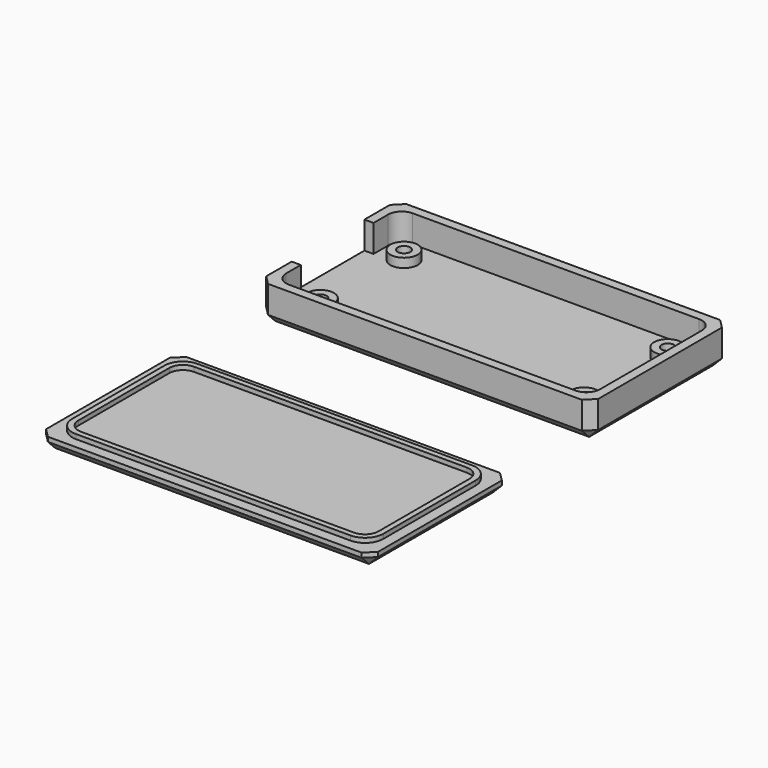
from build123d import *

# Parameters (mm, degrees)
F0_W     = 65
F0_H     = 30
F0_R     = 3
F0_R_2   = 1.375
F0_W_2   = 2
F0_H_2   = 20
F1_DEPTH = 2
F2_DEPTH = 4
F3_DEPTH = 8
F4_R     = 3
F5_SIZE  = 1.99999
F6_SIZE  = 1.7
F7_W     = 73
F7_H     = 38
F7_W_2   = 68.4
F7_H_2   = 33.4
F7_W_3   = 66
F7_H_3   = 31
F7_W_4   = 65
F7_H_4   = 30
F8_DEPTH = 3
F9_DEPTH = 4
F10_R    = 3
F11_R    = 4
F12_SIZE = 2


# Not quite as in the source:
# - a fillet or chamfer is up to 0.001 mm smaller than in the source, because OpenCascade refuses the exact size


with BuildPart() as f1:
    # F0 (on Top) → F1 (new body)
    with BuildSketch(Plane.XY):
        Polygon((-34.5, 10), (-34.5, 17), (34.5, 17), (34.5, -17), (-34.5, -17), (-34.5, -10), (-36.5, -10), (-36.5, -19), (36.5, -19), (36.5, 19), (-36.5, 19), (-36.5, 10), align=None)
        Polygon((34.5, 17), (-34.5, 17), (-34.5, 10), (-34.5, -10), (-34.5, -17), (34.5, -17), align=None)
        Rectangle(F0_W, F0_H, mode=Mode.SUBTRACT)
        Rectangle(F0_W, F0_H)
        with Locations((-29, -11.5)):
            Circle(F0_R, mode=Mode.SUBTRACT)
        with Locations((29, -11.5)):
            Circle(F0_R, mode=Mode.SUBTRACT)
        with Locations((-29, 11.5)):
            Circle(F0_R, mode=Mode.SUBTRACT)
        with Locations((29, 11.5)):
            Circle(F0_R, mode=Mode.SUBTRACT)
        with Locations((-29, 11.5)):
            Circle(F0_R)
        with Locations((-29, 11.5)):
            Circle(F0_R_2, mode=Mode.SUBTRACT)
        with Locations((29, 11.5)):
            Circle(F0_R)
        with Locations((29, 11.5)):
            Circle(F0_R_2, mode=Mode.SUBTRACT)
        with Locations((29, -11.5)):
            Circle(F0_R)
        with Locations((29, -11.5)):
            Circle(F0_R_2, mode=Mode.SUBTRACT)
        with Locations((-29, -11.5)):
            Circle(F0_R)
        with Locations((-29, -11.5)):
            Circle(F0_R_2, mode=Mode.SUBTRACT)
        with Locations((-35.5, 0)):
            Rectangle(F0_W_2, F0_H_2)
    extrude(amount=F1_DEPTH)

    # F0 (on Top) → F2 (join)
    with BuildSketch(Plane.XY):
        with Locations((-29, -11.5)):
            Circle(F0_R)
        with Locations((-29, -11.5)):
            Circle(F0_R_2, mode=Mode.SUBTRACT)
        with Locations((-29, 11.5)):
            Circle(F0_R)
        with Locations((-29, 11.5)):
            Circle(F0_R_2, mode=Mode.SUBTRACT)
        with Locations((29, -11.5)):
            Circle(F0_R)
        with Locations((29, -11.5)):
            Circle(F0_R_2, mode=Mode.SUBTRACT)
        with Locations((29, 11.5)):
            Circle(F0_R)
        with Locations((29, 11.5)):
            Circle(F0_R_2, mode=Mode.SUBTRACT)
    extrude(amount=F2_DEPTH)

    # F0 (on Top) → F3 (join)
    with BuildSketch(Plane.XY):
        Polygon((-34.5, 10), (-34.5, 17), (34.5, 17), (34.5, -17), (-34.5, -17), (-34.5, -10), (-36.5, -10), (-36.5, -19), (36.5, -19), (36.5, 19), (-36.5, 19), (-36.5, 10), align=None)
    extrude(amount=F3_DEPTH)

    # F4
    f4_edges = [f1.edges().sort_by_distance(p)[0] for p in [
        (-34.5, 17, 5),
        (-34.5, -17, 5),
        (34.5, -17, 5),
        (34.5, 17, 5),
    ]]
    fillet(f4_edges, radius=F4_R)

    # F5 (size 2 in the source; OpenCascade refuses exactly that, so slightly less here)
    f5_edges = [f1.edges().sort_by_distance(p)[0] for p in [
        (36.5, -19, 4),
        (36.5, 19, 4),
        (-36.5, 19, 4),
        (-36.5, -19, 4),
        (0, -19, 0),
        (-36.5, 0, 0),
        (0, 19, 0),
        (36.5, 0, 0),
    ]]
    chamfer(f5_edges, length=F5_SIZE)

    # F6
    f6_edges = [f1.edges().sort_by_distance(p)[0] for p in [
        (27.625, 11.5, 0),
        (27.625, -11.5, 0),
        (-30.375, -11.5, 0),
        (-30.375, 11.5, 0),
    ]]
    chamfer(f6_edges, length=F6_SIZE)


with BuildPart() as f8:
    # F7 (on Top) → F8 (new body)
    with BuildSketch(Plane.XY):
        with Locations((0, -60.494761914)):
            Rectangle(F7_W, F7_H)
        with Locations((0, -60.494761914)):
            Rectangle(F7_W_2, F7_H_2, mode=Mode.SUBTRACT)
        with Locations((0, -60.494761914)):
            Rectangle(F7_W_2, F7_H_2)
        with Locations((0, -60.494761914)):
            Rectangle(F7_W_3, F7_H_3, mode=Mode.SUBTRACT)
        with Locations((0, -60.494761914)):
            Rectangle(F7_W_3, F7_H_3)
        with Locations((0, -60.494761914)):
            Rectangle(F7_W_4, F7_H_4, mode=Mode.SUBTRACT)
        with Locations((0, -60.494761914)):
            Rectangle(F7_W_4, F7_H_4)
    extrude(amount=F8_DEPTH)

    # F7 (on Top) → F9 (join)
    with BuildSketch(Plane.XY):
        with Locations((0, -60.494761914)):
            Rectangle(F7_W_2, F7_H_2)
        with Locations((0, -60.494761914)):
            Rectangle(F7_W_3, F7_H_3, mode=Mode.SUBTRACT)
    extrude(amount=F9_DEPTH)

    # F10
    f10_edges = [f8.edges().sort_by_distance(p)[0] for p in [
        (33, -44.994762, 3.5),
        (-33, -44.994762, 3.5),
        (-33, -75.994762, 3.5),
        (33, -75.994762, 3.5),
    ]]
    fillet(f10_edges, radius=F10_R)

    # F11
    f11_edges = [f8.edges().sort_by_distance(p)[0] for p in [
        (-34.2, -43.794762, 3.5),
        (-34.2, -77.194762, 3.5),
        (34.2, -77.194762, 3.5),
        (34.2, -43.794762, 3.5),
    ]]
    fillet(f11_edges, radius=F11_R)

    # F12
    f12_edges = [f8.edges().sort_by_distance(p)[0] for p in [
        (36.5, -79.494762, 1.5),
        (36.5, -41.494762, 1.5),
        (-36.5, -41.494762, 1.5),
        (-36.5, -79.494762, 1.5),
        (-36.5, -60.494762, 0),
        (36.5, -60.494762, 0),
        (0, -41.494762, 0),
        (0, -79.494762, 0),
    ]]
    chamfer(f12_edges, length=F12_SIZE)


solid = Compound([f1.part, f8.part])
